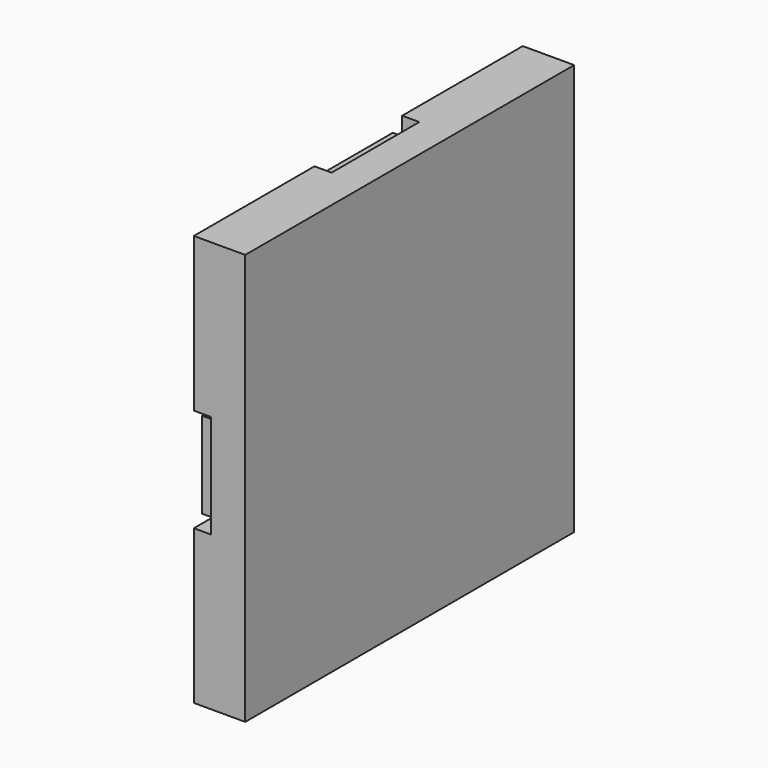
from build123d import *

# Parameters (mm, degrees)
F0_W     = 76.2
F0_H     = 76.2
F0_R     = 24.13
F0_R_2   = 13.97
F1_DEPTH = 6.35
F3_DEPTH = 3.175
F5_DEPTH = 3.175


# Not quite as in the source:
# - after a boolean that leaves OpenCascade's solid faulty, fix() repairs it


with BuildPart() as f1:
    # F0 (on Right) → F1 (new body)
    with BuildSketch(Plane.YZ):
        Rectangle(F0_W, F0_H)
        Circle(F0_R, mode=Mode.SUBTRACT)
        Circle(F0_R)
        Circle(F0_R_2, mode=Mode.SUBTRACT)
        Circle(F0_R_2)
    extrude(amount=F1_DEPTH)

    # F0 (on Right) → F3 (cut)
    with BuildSketch(Plane.YZ):
        Circle(F0_R)
        Circle(F0_R_2, mode=Mode.SUBTRACT)
    extrude(amount=F3_DEPTH, mode=Mode.SUBTRACT)

    # F4 (on face) → F5 (join)
    with BuildSketch(Plane.YZ):
        with BuildLine():
            Line((38.1, 9.5882897328), (38.1, 38.1))
            Line((38.1, 38.1), (10.16, 38.1))
            Line((10.16, 38.1), (10.16, 21.8867836833))
            ThreePointArc((10.16, 21.8867836833), (17.2825787445, 16.8395181624), (22.1432066332, 9.5882897328))
            Line((22.1432066332, 9.5882897328), (38.1, 9.5882897328))
        make_face()
        with BuildLine():
            Line((38.1, -38.1), (38.1, -9.5882897328))
            Line((38.1, -9.5882897328), (22.1432066332, -9.5882897328))
            ThreePointArc((22.1432066332, -9.5882897328), (17.2825787445, -16.8395181624), (10.16, -21.8867836833))
            Line((10.16, -21.8867836833), (10.16, -38.1))
            Line((10.16, -38.1), (38.1, -38.1))
        make_face()
        with BuildLine():
            Line((-10.16, 21.8867836833), (-10.16, 38.1))
            Line((-10.16, 38.1), (-38.1, 38.1))
            Line((-38.1, 38.1), (-38.1, 9.5882897328))
            Line((-38.1, 9.5882897328), (-22.1432066332, 9.5882897328))
            ThreePointArc((-22.1432066332, 9.5882897328), (-17.2825787445, 16.8395181624), (-10.16, 21.8867836833))
        make_face()
        with BuildLine():
            Line((-38.1, -9.5882897328), (-38.1, -38.1))
            Line((-38.1, -38.1), (-10.16, -38.1))
            Line((-10.16, -38.1), (-10.16, -21.8867836833))
            ThreePointArc((-10.16, -21.8867836833), (-17.2825787445, -16.8395181624), (-22.1432066332, -9.5882897328))
            Line((-22.1432066332, -9.5882897328), (-38.1, -9.5882897328))
        make_face()
        with BuildLine():
            Line((36.195, -8.001), (36.195, 8.001))
            Line((36.195, 8.001), (22.7649049855, 8.001))
            ThreePointArc((22.7649049855, 8.001), (24.13, 0), (22.7649049855, -8.001))
            Line((22.7649049855, -8.001), (36.195, -8.001))
        make_face()
        with BuildLine():
            Line((-22.7649049855, 8.001), (-36.195, 8.001))
            Line((-36.195, 8.001), (-36.195, -8.001))
            Line((-36.195, -8.001), (-22.7649049855, -8.001))
            ThreePointArc((-22.7649049855, -8.001), (-24.13, 0), (-22.7649049855, 8.001))
        make_face()
        with BuildLine():
            Line((8.001, 22.7649049855), (8.001, 36.195))
            Line((8.001, 36.195), (-8.001, 36.195))
            Line((-8.001, 36.195), (-8.001, 22.7649049855))
            ThreePointArc((-8.001, 22.7649049855), (0, 24.13), (8.001, 22.7649049855))
        make_face()
        with BuildLine():
            Line((-8.001, -36.195), (8.001, -36.195))
            Line((8.001, -36.195), (8.001, -22.7649049855))
            ThreePointArc((8.001, -22.7649049855), (0, -24.13), (-8.001, -22.7649049855))
            Line((-8.001, -22.7649049855), (-8.001, -36.195))
        make_face()
    extrude(amount=-F5_DEPTH)

    add(f1.part.fix(), mode=Mode.REPLACE)


solid = f1.part
